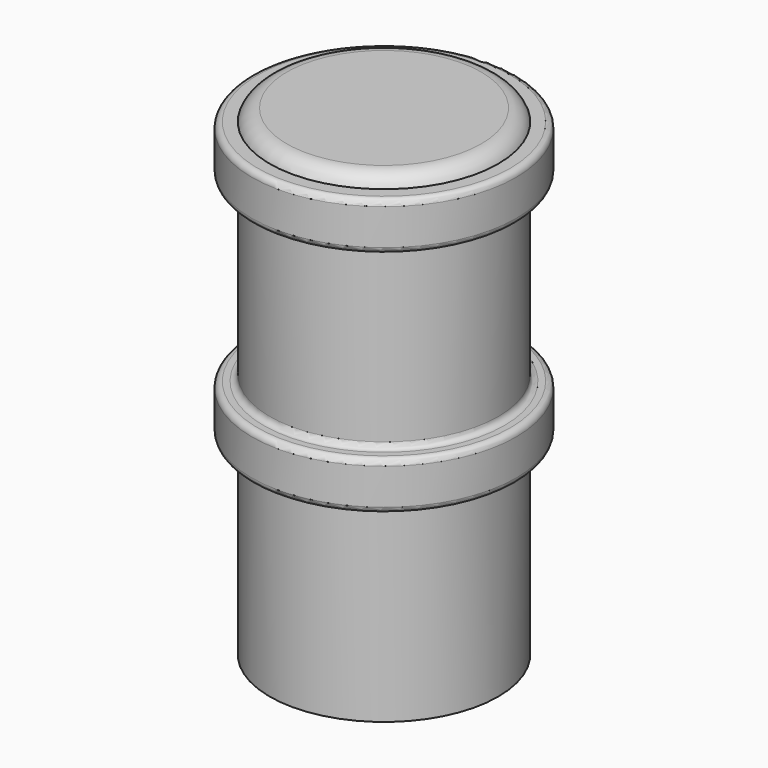
from build123d import *

# Parameters (mm, degrees)
F0_R      = 9.5
F1_DEPTH  = 40
F2_R      = 8.65
F3_DEPTH  = 37.5
F5_R      = 11
F6_DEPTH  = 4
F8_R      = 11
F9_DEPTH  = 4
F11_R     = 0.5
F12_R     = 0.5
F13_R     = 0.5
F14_R     = 0.5
F15_R     = 0.5
F16_R     = 8.65
F17_DEPTH = 39


# Not quite as in the source:
# - a fillet or chamfer that OpenCascade refuses, or shapes differently, is made with other operations: its cross-section is extruded or revolved along the edge and cut away or added


with BuildPart() as f1:
    # F0 (on Top) → F1 (new body)
    with BuildSketch(Plane.XY):
        Circle(F0_R)
    extrude(amount=F1_DEPTH)

    # F2 (on face) → F3 (cut)
    with BuildSketch(Plane(origin=(0, 0, 0), x_dir=(1, 0, 0), z_dir=(0, 0, -1))):
        Circle(F2_R)
    extrude(amount=-F3_DEPTH, mode=Mode.SUBTRACT)

    # F5 (on offset) → F6 (join)
    with BuildSketch(Plane.XY.offset(39)):
        Circle(F5_R)
    extrude(amount=-F6_DEPTH)

    # F8 (on offset) → F9 (join)
    with BuildSketch(Plane.XY.offset(20)):
        Circle(F8_R)
    extrude(amount=-F9_DEPTH)

    # F10: fillet of radius 1.5 on 1 edges, made by hand

    # F10_s1 → F10_t2 (revolve, cut)
    with BuildSketch(Plane.XZ):
        with BuildLine():
            ThreePointArc((9.5, 39), (8.9518118414, 39.7247448714), (8.0857864376, 40))
            Line((8.0857864376, 40), (9.5, 40))
            Line((9.5, 40), (9.5, 39))
        make_face()
    revolve(axis=Axis((0, 0, 40), (0, 0, 1)), mode=Mode.SUBTRACT)

    # F11
    f11_edges = [f1.edges().sort_by_distance(p)[0] for p in [
        (11, 0, 37),
        (-11, 0, 39),
        (-11, 0, 35),
    ]]
    fillet(f11_edges, radius=F11_R)

    # F12
    f12_edges = [f1.edges().sort_by_distance(p)[0] for p in [
        (-9.5, 0, 35),
    ]]
    fillet(f12_edges, radius=F12_R)

    # F13
    f13_edges = [f1.edges().sort_by_distance(p)[0] for p in [
        (11, 0, 18),
        (-11, 0, 20),
        (-11, 0, 16),
    ]]
    fillet(f13_edges, radius=F13_R)

    # F14
    f14_edges = [f1.edges().sort_by_distance(p)[0] for p in [
        (-9.5, 0, 20),
    ]]
    fillet(f14_edges, radius=F14_R)

    # F15
    f15_edges = [f1.edges().sort_by_distance(p)[0] for p in [
        (-9.5, 0, 16),
    ]]
    fillet(f15_edges, radius=F15_R)

    # F16 (on face) → F17 (cut)
    with BuildSketch(Plane(origin=(0, 0, 0), x_dir=(1, 0, 0), z_dir=(0, 0, -1))):
        Circle(F16_R)
    extrude(amount=-F17_DEPTH, mode=Mode.SUBTRACT)


solid = f1.part
